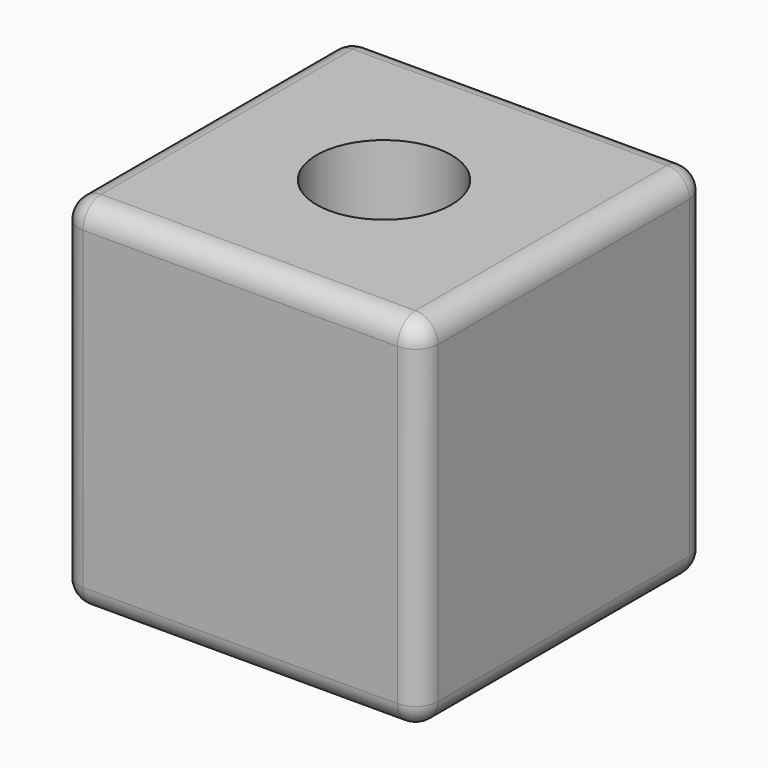
from build123d import *

# Parameters (mm, degrees)
F0_W         = 80
F0_H         = 80
F1_DEPTH     = 40
F2_R         = 5
F3_T1_DEPTH  = 70
F3_S5_W      = 5
F3_S5_H      = 5
F3_T6_DEPTH  = 5
F3_S11_W     = 5
F3_S11_H     = 5
F3_T12_DEPTH = 5
F4_R         = 15
F5_DEPTH     = 80.001


# Not quite as in the source:
# - a fillet or chamfer that OpenCascade refuses, or shapes differently, is made with other operations: its cross-section is extruded or revolved along the edge and cut away or added


with BuildPart() as f1:
    # F0 (on Top) → F1 (new body, symmetric)
    with BuildSketch(Plane.XY):
        Rectangle(F0_W, F0_H)
    extrude(amount=F1_DEPTH, both=True)

    # F2
    f2_edges = [f1.edges().sort_by_distance(p)[0] for p in [
        (0, 40, 40),
        (0, -40, 40),
        (40, 0, 40),
        (-40, 40, 0),
        (-40, 0, -40),
        (-40, -40, 0),
        (-40, 0, 40),
        (40, 40, 0),
        (40, 0, -40),
        (40, -40, 0),
        (0, -40, -40),
    ]]
    fillet(f2_edges, radius=F2_R)

    # F3: fillet of radius 5 on 1 edges, made by hand

    # F3_s2 → F3_t1 (cut)
    with BuildSketch(Plane.YZ.offset(-35)):
        with BuildLine():
            ThreePointArc((35, -40), (38.5355339059, -38.5355339059), (40, -35))
            Line((40, -35), (40, -40))
            Line((40, -40), (35, -40))
        make_face()
    extrude(amount=F3_T1_DEPTH, mode=Mode.SUBTRACT)


with BuildPart() as f3_tool4:
    # F3_s5 → F3_t6 (new body)
    with BuildSketch(Plane.XY.offset(-35)):
        with Locations((37.5, 37.5)):
            Rectangle(F3_S5_W, F3_S5_H)
    extrude(amount=-F3_T6_DEPTH)

    # F3_s7 → F3_t8 (revolve, cut)
    with BuildSketch(Plane(origin=(35, 35, -35), x_dir=(-0.7071067812, -0.7071067812, 0), z_dir=(0.7071067812, -0.7071067812, 0))):
        with BuildLine():
            ThreePointArc((0, -5), (5, 0), (0, 5))
            Line((0, 5), (0, -5))
        make_face()
    revolve(axis=Axis((35, 35, -35), (0, 0, -1)), mode=Mode.SUBTRACT)


with BuildPart() as f1_1:
    add(f1.part)

    # F3_t3: cut F3_tool4
    add(f3_tool4.part, mode=Mode.SUBTRACT)


with BuildPart() as f3_tool10:
    # F3_s11 → F3_t12 (new body)
    with BuildSketch(Plane.XY.offset(-35)):
        with Locations((-37.5, 37.5)):
            Rectangle(F3_S11_W, F3_S11_H)
    extrude(amount=-F3_T12_DEPTH)

    # F3_s13 → F3_t14 (revolve, cut)
    with BuildSketch(Plane(origin=(-35, 35, -35), x_dir=(0.7071067812, -0.7071067812, 0), z_dir=(0.7071067812, 0.7071067812, 0))):
        with BuildLine():
            ThreePointArc((0, -5), (5, 0), (0, 5))
            Line((0, 5), (0, -5))
        make_face()
    revolve(axis=Axis((-35, 35, -35), (0, 0, -1)), mode=Mode.SUBTRACT)


with BuildPart() as f1_2:
    add(f1_1.part)

    # F3_t9: cut F3_tool10
    add(f3_tool10.part, mode=Mode.SUBTRACT)

    # F4 (on face) → F5 (cut, through all)
    with BuildSketch(Plane.XY.offset(40)):
        Circle(F4_R)
    extrude(amount=-F5_DEPTH, mode=Mode.SUBTRACT)


solid = f1_2.part
